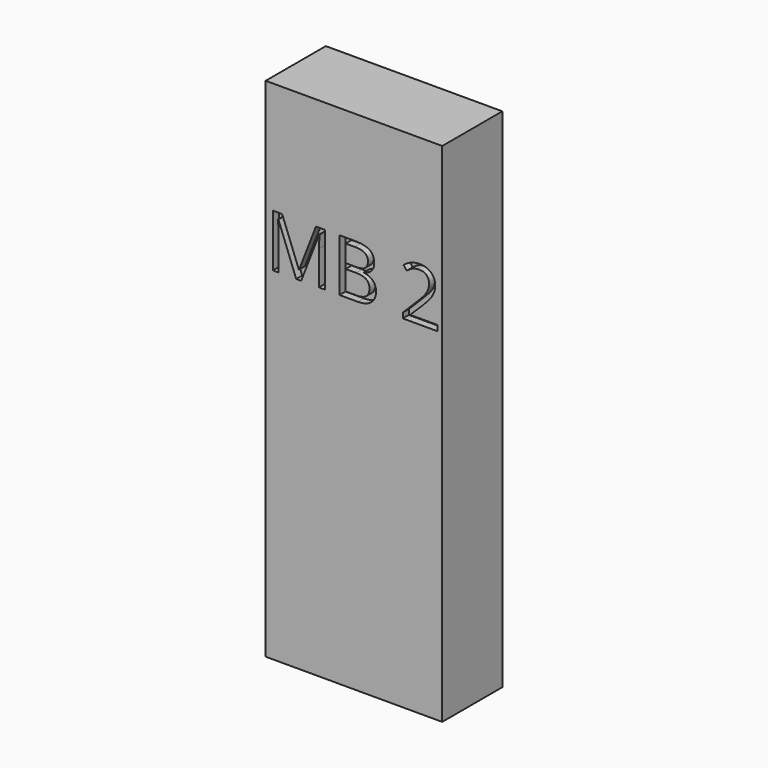
from build123d import *

# Parameters (mm, degrees)
F0_W         = 596.9
F0_H         = 1714.5
F1_DEPTH     = 127
F2_TEXT_SIZE = 249.3739800248
F3_DEPTH     = 25.4


# Not quite as in the source:
# - Text() gives the source's letters only with a copy of the font that has no kerning and outlines rounded to 1/6400 em; it was checked with that copy


with BuildPart() as f1:
    # F0 (on Front) → F1 (new body, symmetric)
    with BuildSketch(Plane.XZ):
        Rectangle(F0_W, F0_H)
    extrude(amount=F1_DEPTH, both=True)

    # F2 (on face) → F3 (cut)
    with BuildSketch(Plane.XZ.offset(127)):
        with Locations((-298.45, 300.5997377254)):
            Text('MB 2', F2_TEXT_SIZE, font='Open Sans', text_align=(TextAlign.LEFT, TextAlign.BOTTOM))
    extrude(amount=-F3_DEPTH, mode=Mode.SUBTRACT)


solid = f1.part
